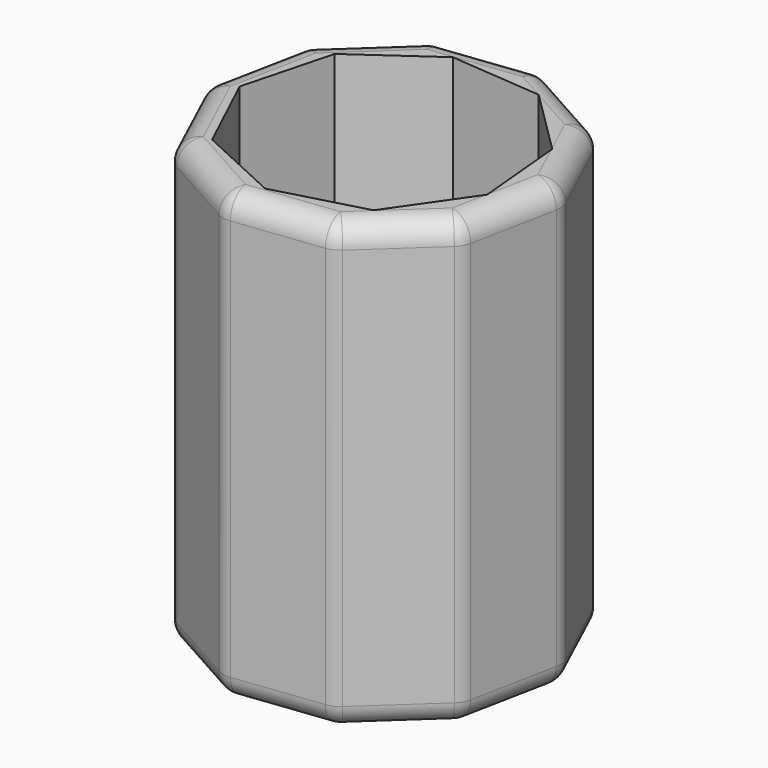
from build123d import *

# Parameters (mm, degrees)
F1_DEPTH      = 100
F2_T1_DEPTH   = 90
F2_T3_DEPTH   = 19.5857421182
F2_T5_DEPTH   = 19.5857421182
F2_T7_DEPTH   = 19.5857421182
F2_T9_DEPTH   = 19.5857421182
F2_T11_DEPTH  = 19.5857421182
F2_T13_DEPTH  = 19.5857421182
F2_T15_DEPTH  = 19.5857421182
F2_T17_DEPTH  = 19.5857421182
F2_T19_DEPTH  = 19.5857421182
F2_T21_DEPTH  = 19.5857421182
F2_T26_DEPTH  = 5
F2_T32_DEPTH  = 5
F2_T38_DEPTH  = 5
F2_T44_DEPTH  = 5
F2_T50_DEPTH  = 5
F2_T56_DEPTH  = 5
F2_T62_DEPTH  = 5
F2_T68_DEPTH  = 5
F2_T74_DEPTH  = 5
F2_T80_DEPTH  = 5
F2_T86_DEPTH  = 5
F2_T92_DEPTH  = 5
F2_T98_DEPTH  = 5
F2_T104_DEPTH = 5
F2_T110_DEPTH = 5
F2_T116_DEPTH = 5
F2_T122_DEPTH = 5
F2_T128_DEPTH = 5
F2_T134_DEPTH = 5
F2_T140_DEPTH = 5


# Not quite as in the source:
# - a fillet or chamfer that OpenCascade refuses, or shapes differently, is made with other operations: its cross-section is extruded or revolved along the edge and cut away or added


with BuildPart() as f1:
    # F0 (on Top) → F1 (new body)
    with BuildSketch(Plane.XY):
        Polygon((27.1144770649, 25.0985702318), (7.1835033032, 36.2426595944), (-15.491324562, 33.5432848347), (-32.2489929753, 18.0315153624), (-36.688642175, -4.3676801097), (-27.1144770649, -25.0985702318), (-7.1835033032, -36.2426595944), (15.491324562, -33.5432848347), (32.2489929753, -18.0315153624), (36.688642175, 4.3676801097), align=None)
        Polygon((-24.8698702516, 17.2562639713), (-7.9593132371, 29.2051095764), (12.675494899, 27.4885598321), (27.3792980994, 12.909807441), (29.272023432, -7.7095873283), (17.4680436786, -24.7215805041), (-2.5094278478, -30.1660714123), (-21.312710195, -21.4955222482), (-30.1435385776, -2.766979328), align=None, mode=Mode.SUBTRACT)
    extrude(amount=F1_DEPTH)

    # F2: fillet of radius 5 on 30 edges, made by hand

    # F2_s2 → F2_t1 (cut)
    with BuildSketch(Plane.XY.offset(5)):
        with BuildLine():
            ThreePointArc((-8.6014983146, -35.4498100673), (-7.1334759697, -35.9902585663), (-5.5702959817, -36.0506117803))
            Line((-5.5702959817, -36.0506117803), (-7.1835033032, -36.2426595944))
            Line((-7.1835033032, -36.2426595944), (-8.6014983146, -35.4498100673))
        make_face()
        with BuildLine():
            ThreePointArc((13.8781172405, -33.7353326487), (15.383439923, -33.3096827847), (16.6835538277, -32.4396954169))
            Line((16.6835538277, -32.4396954169), (15.491324562, -33.5432848347))
            Line((15.491324562, -33.5432848347), (13.8781172405, -33.7353326487))
        make_face()
        with BuildLine():
            ThreePointArc((32.5648531281, -16.4379179889), (32.024404629, -17.9059403338), (31.0567637096, -19.1351047802))
            Line((31.0567637096, -19.1351047802), (32.2489929753, -18.0315153624))
            Line((32.2489929753, -18.0315153624), (32.5648531281, -16.4379179889))
        make_face()
        with BuildLine():
            ThreePointArc((36.3727820222, 2.7740827361), (36.4331352362, 4.3372627241), (36.0074853722, 5.8425854066))
            Line((36.0074853722, 5.8425854066), (36.688642175, 4.3676801097))
            Line((36.688642175, 4.3676801097), (36.3727820222, 2.7740827361))
        make_face()
        with BuildLine():
            ThreePointArc((-27.7956338677, -23.6236649348), (-26.9256464999, -24.9237788395), (-25.6964820535, -25.8914197589))
            Line((-25.6964820535, -25.8914197589), (-27.1144770649, -25.0985702318))
            Line((-27.1144770649, -25.0985702318), (-27.7956338677, -23.6236649348))
        make_face()
        with BuildLine():
            ThreePointArc((-36.3727820222, -2.7740827361), (-36.4331352362, -4.3372627241), (-36.0074853722, -5.8425854066))
            Line((-36.0074853722, -5.8425854066), (-36.688642175, -4.3676801097))
            Line((-36.688642175, -4.3676801097), (-36.3727820222, -2.7740827361))
        make_face()
        with BuildLine():
            ThreePointArc((-31.0567637096, 19.1351047802), (-32.024404629, 17.9059403338), (-32.5648531281, 16.4379179889))
            Line((-32.5648531281, 16.4379179889), (-32.2489929753, 18.0315153624))
            Line((-32.2489929753, 18.0315153624), (-31.0567637096, 19.1351047802))
        make_face()
        with BuildLine():
            ThreePointArc((-13.8781172405, 33.7353326487), (-15.383439923, 33.3096827847), (-16.6835538277, 32.4396954169))
            Line((-16.6835538277, 32.4396954169), (-15.491324562, 33.5432848347))
            Line((-15.491324562, 33.5432848347), (-13.8781172405, 33.7353326487))
        make_face()
        with BuildLine():
            ThreePointArc((8.6014983146, 35.4498100673), (7.1334759697, 35.9902585663), (5.5702959817, 36.0506117803))
            Line((5.5702959817, 36.0506117803), (7.1835033032, 36.2426595944))
            Line((7.1835033032, 36.2426595944), (8.6014983146, 35.4498100673))
        make_face()
        with BuildLine():
            ThreePointArc((27.7956338677, 23.6236649348), (26.9256464999, 24.9237788395), (25.6964820535, 25.8914197589))
            Line((25.6964820535, 25.8914197589), (27.1144770649, 25.0985702318))
            Line((27.1144770649, 25.0985702318), (27.7956338677, 23.6236649348))
        make_face()
    extrude(amount=F2_T1_DEPTH, mode=Mode.SUBTRACT)

    # F2_s4 → F2_t3 (cut)
    with BuildSketch(Plane(origin=(-9.7242066111, -1.1576395658, 0), x_dir=(0, 0, 1), z_dir=(0.9929883231, 0.1182124791, 0))):
        with BuildLine():
            ThreePointArc((5, 35.1393580403), (1.4644660941, 33.6748919462), (0, 30.1393580403))
            Line((0, 30.1393580403), (0, 35.1393580403))
            Line((0, 35.1393580403), (5, 35.1393580403))
        make_face()
        with BuildLine():
            ThreePointArc((95, 35.1393580403), (98.5355339059, 33.6748919462), (100, 30.1393580403))
            Line((100, 30.1393580403), (100, 35.1393580403))
            Line((100, 35.1393580403), (95, 35.1393580403))
        make_face()
    extrude(amount=F2_T3_DEPTH, mode=Mode.SUBTRACT)

    # F2_s6 → F2_t5 (cut)
    with BuildSketch(Plane(origin=(-7.186604941, -6.6522953184, 0), x_dir=(0, 0, 1), z_dir=(0.7338608767, 0.6792997966, 0))):
        with BuildLine():
            ThreePointArc((5, 35.1393580403), (1.4644660941, 33.6748919462), (0, 30.1393580403))
            Line((0, 30.1393580403), (0, 35.1393580403))
            Line((0, 35.1393580403), (5, 35.1393580403))
        make_face()
        with BuildLine():
            ThreePointArc((95, 35.1393580403), (98.5355339059, 33.6748919462), (100, 30.1393580403))
            Line((100, 30.1393580403), (100, 35.1393580403))
            Line((100, 35.1393580403), (95, 35.1393580403))
        make_face()
    extrude(amount=F2_T5_DEPTH, mode=Mode.SUBTRACT)

    # F2_s8 → F2_t7 (cut)
    with BuildSketch(Plane(origin=(-1.9039644471, -9.6060003625, 0), x_dir=(0, 0, 1), z_dir=(0.1944235185, 0.9809176803, 0))):
        with BuildLine():
            ThreePointArc((5, 35.1393580403), (1.4644660941, 33.6748919462), (0, 30.1393580403))
            Line((0, 30.1393580403), (0, 35.1393580403))
            Line((0, 35.1393580403), (5, 35.1393580403))
        make_face()
        with BuildLine():
            ThreePointArc((95, 35.1393580403), (98.5355339059, 33.6748919462), (100, 30.1393580403))
            Line((100, 30.1393580403), (100, 35.1393580403))
            Line((100, 35.1393580403), (95, 35.1393580403))
        make_face()
    extrude(amount=F2_T7_DEPTH, mode=Mode.SUBTRACT)

    # F2_s10 → F2_t9 (cut)
    with BuildSketch(Plane(origin=(-8.5474918695, 4.7791951542, 0), x_dir=(0, 0, 1), z_dir=(0.8728279805, -0.4880279874, 0))):
        with BuildLine():
            ThreePointArc((5, 35.1393580403), (1.4644660941, 33.6748919462), (0, 30.1393580403))
            Line((0, 30.1393580403), (0, 35.1393580403))
            Line((0, 35.1393580403), (5, 35.1393580403))
        make_face()
        with BuildLine():
            ThreePointArc((95, 35.1393580403), (98.5355339059, 33.6748919462), (100, 30.1393580403))
            Line((100, 30.1393580403), (100, 35.1393580403))
            Line((100, 35.1393580403), (95, 35.1393580403))
        make_face()
    extrude(amount=F2_T9_DEPTH, mode=Mode.SUBTRACT)

    # F2_s12 → F2_t11 (cut)
    with BuildSketch(Plane(origin=(-4.1059257522, 8.8905397641, 0), x_dir=(0, 0, 1), z_dir=(0.4192770156, -0.9078583503, 0))):
        with BuildLine():
            ThreePointArc((5, 35.1393580403), (1.4644660941, 33.6748919462), (0, 30.1393580403))
            Line((0, 30.1393580403), (0, 35.1393580403))
            Line((0, 35.1393580403), (5, 35.1393580403))
        make_face()
        with BuildLine():
            ThreePointArc((95, 35.1393580403), (98.5355339059, 33.6748919462), (100, 30.1393580403))
            Line((100, 30.1393580403), (100, 35.1393580403))
            Line((100, 35.1393580403), (95, 35.1393580403))
        make_face()
    extrude(amount=F2_T11_DEPTH, mode=Mode.SUBTRACT)

    # F2_s14 → F2_t13 (cut)
    with BuildSketch(Plane(origin=(1.9039644471, 9.6060003625, 0), x_dir=(0, 0, 1), z_dir=(-0.1944235185, -0.9809176803, 0))):
        with BuildLine():
            ThreePointArc((5, 35.1393580403), (1.4644660941, 33.6748919462), (0, 30.1393580403))
            Line((0, 30.1393580403), (0, 35.1393580403))
            Line((0, 35.1393580403), (5, 35.1393580403))
        make_face()
        with BuildLine():
            ThreePointArc((95, 35.1393580403), (98.5355339059, 33.6748919462), (100, 30.1393580403))
            Line((100, 30.1393580403), (100, 35.1393580403))
            Line((100, 35.1393580403), (95, 35.1393580403))
        make_face()
    extrude(amount=F2_T13_DEPTH, mode=Mode.SUBTRACT)

    # F2_s16 → F2_t15 (cut)
    with BuildSketch(Plane(origin=(7.186604941, 6.6522953184, 0), x_dir=(0, 0, 1), z_dir=(-0.7338608767, -0.6792997966, 0))):
        with BuildLine():
            ThreePointArc((5, 35.1393580403), (1.4644660941, 33.6748919462), (0, 30.1393580403))
            Line((0, 30.1393580403), (0, 35.1393580403))
            Line((0, 35.1393580403), (5, 35.1393580403))
        make_face()
        with BuildLine():
            ThreePointArc((95, 35.1393580403), (98.5355339059, 33.6748919462), (100, 30.1393580403))
            Line((100, 30.1393580403), (100, 35.1393580403))
            Line((100, 35.1393580403), (95, 35.1393580403))
        make_face()
    extrude(amount=F2_T15_DEPTH, mode=Mode.SUBTRACT)

    # F2_s18 → F2_t17 (cut)
    with BuildSketch(Plane(origin=(9.7242066111, 1.1576395658, 0), x_dir=(0, 0, 1), z_dir=(-0.9929883231, -0.1182124791, 0))):
        with BuildLine():
            ThreePointArc((5, 35.1393580403), (1.4644660941, 33.6748919462), (0, 30.1393580403))
            Line((0, 30.1393580403), (0, 35.1393580403))
            Line((0, 35.1393580403), (5, 35.1393580403))
        make_face()
        with BuildLine():
            ThreePointArc((95, 35.1393580403), (98.5355339059, 33.6748919462), (100, 30.1393580403))
            Line((100, 30.1393580403), (100, 35.1393580403))
            Line((100, 35.1393580403), (95, 35.1393580403))
        make_face()
    extrude(amount=F2_T17_DEPTH, mode=Mode.SUBTRACT)

    # F2_s20 → F2_t19 (cut)
    with BuildSketch(Plane(origin=(8.5474918695, -4.7791951542, 0), x_dir=(0, 0, 1), z_dir=(-0.8728279805, 0.4880279874, 0))):
        with BuildLine():
            ThreePointArc((5, 35.1393580403), (1.4644660941, 33.6748919462), (0, 30.1393580403))
            Line((0, 30.1393580403), (0, 35.1393580403))
            Line((0, 35.1393580403), (5, 35.1393580403))
        make_face()
        with BuildLine():
            ThreePointArc((95, 35.1393580403), (98.5355339059, 33.6748919462), (100, 30.1393580403))
            Line((100, 30.1393580403), (100, 35.1393580403))
            Line((100, 35.1393580403), (95, 35.1393580403))
        make_face()
    extrude(amount=F2_T19_DEPTH, mode=Mode.SUBTRACT)

    # F2_s22 → F2_t21 (cut)
    with BuildSketch(Plane(origin=(4.1059257522, -8.8905397641, 0), x_dir=(0, 0, 1), z_dir=(-0.4192770156, 0.9078583503, 0))):
        with BuildLine():
            ThreePointArc((5, 35.1393580403), (1.4644660941, 33.6748919462), (0, 30.1393580403))
            Line((0, 30.1393580403), (0, 35.1393580403))
            Line((0, 35.1393580403), (5, 35.1393580403))
        make_face()
        with BuildLine():
            ThreePointArc((95, 35.1393580403), (98.5355339059, 33.6748919462), (100, 30.1393580403))
            Line((100, 30.1393580403), (100, 35.1393580403))
            Line((100, 35.1393580403), (95, 35.1393580403))
        make_face()
    extrude(amount=F2_T21_DEPTH, mode=Mode.SUBTRACT)


with BuildPart() as f2_tool24:
    # F2_s25 → F2_t26 (new body)
    with BuildSketch(Plane.XY.offset(5)):
        Polygon((-6.1613583774, -31.0856701649), (-8.6014983146, -35.4498100673), (-7.1835033032, -36.2426595944), (-5.5702959817, -36.0506117803), align=None)
    extrude(amount=-F2_T26_DEPTH)

    # F2_s27 → F2_t28 (revolve, cut)
    with BuildSketch(Plane(origin=(-6.1613583774, -31.0856701649, 5), x_dir=(0.1944235185, 0.9809176803, 0), z_dir=(-0.9809176803, 0.1944235185, 0))):
        with BuildLine():
            ThreePointArc((0, -5), (5, 0), (0, 5))
            Line((0, 5), (0, -5))
        make_face()
    revolve(axis=Axis((-6.1613583774, -31.0856701649, 5), (0, 0, -1)), mode=Mode.SUBTRACT)


with BuildPart() as f1_1:
    add(f1.part)

    # F2_t23: cut F2_tool24
    add(f2_tool24.part, mode=Mode.SUBTRACT)


with BuildPart() as f2_tool30:
    # F2_s31 → F2_t32 (new body)
    with BuildSketch(Plane.XY.offset(95)):
        Polygon((-6.1613583774, -31.0856701649), (-8.6014983146, -35.4498100673), (-7.1835033032, -36.2426595944), (-5.5702959817, -36.0506117803), align=None)
    extrude(amount=F2_T32_DEPTH)

    # F2_s33 → F2_t34 (revolve, cut)
    with BuildSketch(Plane(origin=(-6.1613583774, -31.0856701649, 95), x_dir=(0.1944235185, 0.9809176803, 0), z_dir=(0.9809176803, -0.1944235185, 0))):
        with BuildLine():
            ThreePointArc((0, -5), (5, 0), (0, 5))
            Line((0, 5), (0, -5))
        make_face()
    revolve(axis=Axis((-6.1613583774, -31.0856701649, 95), (0, 0, 1)), mode=Mode.SUBTRACT)


with BuildPart() as f1_2:
    add(f1_1.part)

    # F2_t29: cut F2_tool30
    add(f2_tool30.part, mode=Mode.SUBTRACT)


with BuildPart() as f2_tool36:
    # F2_s37 → F2_t38 (new body)
    with BuildSketch(Plane.XY.offset(5)):
        Polygon((13.2870548448, -28.7703910333), (13.8781172405, -33.7353326487), (15.491324562, -33.5432848347), (16.6835538277, -32.4396954169), align=None)
    extrude(amount=-F2_T38_DEPTH)

    # F2_s39 → F2_t40 (revolve, cut)
    with BuildSketch(Plane(origin=(13.2870548448, -28.7703910333, 5), x_dir=(-0.4192770156, 0.9078583503, 0), z_dir=(-0.9078583503, -0.4192770156, 0))):
        with BuildLine():
            ThreePointArc((0, -5), (5, 0), (0, 5))
            Line((0, 5), (0, -5))
        make_face()
    revolve(axis=Axis((13.2870548448, -28.7703910333, 5), (0, 0, -1)), mode=Mode.SUBTRACT)


with BuildPart() as f1_3:
    add(f1_2.part)

    # F2_t35: cut F2_tool36
    add(f2_tool36.part, mode=Mode.SUBTRACT)


with BuildPart() as f2_tool42:
    # F2_s43 → F2_t44 (new body)
    with BuildSketch(Plane.XY.offset(95)):
        Polygon((13.2870548448, -28.7703910333), (13.8781172405, -33.7353326487), (15.491324562, -33.5432848347), (16.6835538277, -32.4396954169), align=None)
    extrude(amount=F2_T44_DEPTH)

    # F2_s45 → F2_t46 (revolve, cut)
    with BuildSketch(Plane(origin=(13.2870548448, -28.7703910333, 95), x_dir=(-0.4192770156, 0.9078583503, 0), z_dir=(0.9078583503, 0.4192770156, 0))):
        with BuildLine():
            ThreePointArc((0, -5), (5, 0), (0, 5))
            Line((0, 5), (0, -5))
        make_face()
    revolve(axis=Axis((13.2870548448, -28.7703910333, 95), (0, 0, 1)), mode=Mode.SUBTRACT)


with BuildPart() as f1_4:
    add(f1_3.part)

    # F2_t41: cut F2_tool42
    add(f2_tool42.part, mode=Mode.SUBTRACT)


with BuildPart() as f2_tool48:
    # F2_s49 → F2_t50 (new body)
    with BuildSketch(Plane.XY.offset(5)):
        Polygon((27.6602647267, -15.4658003966), (32.5648531281, -16.4379179889), (32.2489929753, -18.0315153624), (31.0567637096, -19.1351047802), align=None)
    extrude(amount=-F2_T50_DEPTH)

    # F2_s51 → F2_t52 (revolve, cut)
    with BuildSketch(Plane(origin=(27.6602647267, -15.4658003966, 5), x_dir=(-0.8728279805, 0.4880279874, 0), z_dir=(-0.4880279874, -0.8728279805, 0))):
        with BuildLine():
            ThreePointArc((0, -5), (5, 0), (0, 5))
            Line((0, 5), (0, -5))
        make_face()
    revolve(axis=Axis((27.6602647267, -15.4658003966, 5), (0, 0, -1)), mode=Mode.SUBTRACT)


with BuildPart() as f1_5:
    add(f1_4.part)

    # F2_t47: cut F2_tool48
    add(f2_tool48.part, mode=Mode.SUBTRACT)


with BuildPart() as f2_tool54:
    # F2_s55 → F2_t56 (new body)
    with BuildSketch(Plane.XY.offset(95)):
        Polygon((27.6602647267, -15.4658003966), (32.5648531281, -16.4379179889), (32.2489929753, -18.0315153624), (31.0567637096, -19.1351047802), align=None)
    extrude(amount=F2_T56_DEPTH)

    # F2_s57 → F2_t58 (revolve, cut)
    with BuildSketch(Plane(origin=(27.6602647267, -15.4658003966, 95), x_dir=(-0.8728279805, 0.4880279874, 0), z_dir=(0.4880279874, 0.8728279805, 0))):
        with BuildLine():
            ThreePointArc((0, -5), (5, 0), (0, 5))
            Line((0, 5), (0, -5))
        make_face()
    revolve(axis=Axis((27.6602647267, -15.4658003966, 95), (0, 0, 1)), mode=Mode.SUBTRACT)


with BuildPart() as f1_6:
    add(f1_5.part)

    # F2_t53: cut F2_tool54
    add(f2_tool54.part, mode=Mode.SUBTRACT)


with BuildPart() as f2_tool60:
    # F2_s61 → F2_t62 (new body)
    with BuildSketch(Plane.XY.offset(5)):
        Polygon((31.4681936208, 3.7462003284), (36.3727820222, 2.7740827361), (36.688642175, 4.3676801097), (36.0074853722, 5.8425854066), align=None)
    extrude(amount=-F2_T62_DEPTH)

    # F2_s63 → F2_t64 (revolve, cut)
    with BuildSketch(Plane(origin=(31.4681936208, 3.7462003284, 5), x_dir=(-0.9929883231, -0.1182124791, 0), z_dir=(0.1182124791, -0.9929883231, 0))):
        with BuildLine():
            ThreePointArc((0, -5), (5, 0), (0, 5))
            Line((0, 5), (0, -5))
        make_face()
    revolve(axis=Axis((31.4681936208, 3.7462003284, 5), (0, 0, -1)), mode=Mode.SUBTRACT)


with BuildPart() as f1_7:
    add(f1_6.part)

    # F2_t59: cut F2_tool60
    add(f2_tool60.part, mode=Mode.SUBTRACT)


with BuildPart() as f2_tool66:
    # F2_s67 → F2_t68 (new body)
    with BuildSketch(Plane.XY.offset(95)):
        Polygon((31.4681936208, 3.7462003284), (36.3727820222, 2.7740827361), (36.688642175, 4.3676801097), (36.0074853722, 5.8425854066), align=None)
    extrude(amount=F2_T68_DEPTH)

    # F2_s69 → F2_t70 (revolve, cut)
    with BuildSketch(Plane(origin=(31.4681936208, 3.7462003284, 95), x_dir=(-0.9929883231, -0.1182124791, 0), z_dir=(-0.1182124791, 0.9929883231, 0))):
        with BuildLine():
            ThreePointArc((0, -5), (5, 0), (0, 5))
            Line((0, 5), (0, -5))
        make_face()
    revolve(axis=Axis((31.4681936208, 3.7462003284, 95), (0, 0, 1)), mode=Mode.SUBTRACT)


with BuildPart() as f1_8:
    add(f1_7.part)

    # F2_t65: cut F2_tool66
    add(f2_tool66.part, mode=Mode.SUBTRACT)


with BuildPart() as f2_tool72:
    # F2_s73 → F2_t74 (new body)
    with BuildSketch(Plane.XY.offset(5)):
        Polygon((-23.2563421164, -21.5272798566), (-27.7956338677, -23.6236649348), (-27.1144770649, -25.0985702318), (-25.6964820535, -25.8914197589), align=None)
    extrude(amount=-F2_T74_DEPTH)

    # F2_s75 → F2_t76 (revolve, cut)
    with BuildSketch(Plane(origin=(-23.2563421164, -21.5272798566, 5), x_dir=(0.7338608767, 0.6792997966, 0), z_dir=(-0.6792997966, 0.7338608767, 0))):
        with BuildLine():
            ThreePointArc((0, -5), (5, 0), (0, 5))
            Line((0, 5), (0, -5))
        make_face()
    revolve(axis=Axis((-23.2563421164, -21.5272798566, 5), (0, 0, -1)), mode=Mode.SUBTRACT)


with BuildPart() as f1_9:
    add(f1_8.part)

    # F2_t71: cut F2_tool72
    add(f2_tool72.part, mode=Mode.SUBTRACT)


with BuildPart() as f2_tool78:
    # F2_s79 → F2_t80 (new body)
    with BuildSketch(Plane.XY.offset(95)):
        Polygon((-23.2563421164, -21.5272798566), (-27.7956338677, -23.6236649348), (-27.1144770649, -25.0985702318), (-25.6964820535, -25.8914197589), align=None)
    extrude(amount=F2_T80_DEPTH)

    # F2_s81 → F2_t82 (revolve, cut)
    with BuildSketch(Plane(origin=(-23.2563421164, -21.5272798566, 95), x_dir=(0.7338608767, 0.6792997966, 0), z_dir=(0.6792997966, -0.7338608767, 0))):
        with BuildLine():
            ThreePointArc((0, -5), (5, 0), (0, 5))
            Line((0, 5), (0, -5))
        make_face()
    revolve(axis=Axis((-23.2563421164, -21.5272798566, 95), (0, 0, 1)), mode=Mode.SUBTRACT)


with BuildPart() as f1_10:
    add(f1_9.part)

    # F2_t77: cut F2_tool78
    add(f2_tool78.part, mode=Mode.SUBTRACT)


with BuildPart() as f2_tool84:
    # F2_s85 → F2_t86 (new body)
    with BuildSketch(Plane.XY.offset(5)):
        Polygon((-31.4681936208, -3.7462003284), (-36.3727820222, -2.7740827361), (-36.688642175, -4.3676801097), (-36.0074853722, -5.8425854066), align=None)
    extrude(amount=-F2_T86_DEPTH)

    # F2_s87 → F2_t88 (revolve, cut)
    with BuildSketch(Plane(origin=(-31.4681936208, -3.7462003284, 5), x_dir=(0.9929883231, 0.1182124791, 0), z_dir=(-0.1182124791, 0.9929883231, 0))):
        with BuildLine():
            ThreePointArc((0, -5), (5, 0), (0, 5))
            Line((0, 5), (0, -5))
        make_face()
    revolve(axis=Axis((-31.4681936208, -3.7462003284, 5), (0, 0, -1)), mode=Mode.SUBTRACT)


with BuildPart() as f1_11:
    add(f1_10.part)

    # F2_t83: cut F2_tool84
    add(f2_tool84.part, mode=Mode.SUBTRACT)


with BuildPart() as f2_tool90:
    # F2_s91 → F2_t92 (new body)
    with BuildSketch(Plane.XY.offset(95)):
        Polygon((-31.4681936208, -3.7462003284), (-36.3727820222, -2.7740827361), (-36.688642175, -4.3676801097), (-36.0074853722, -5.8425854066), align=None)
    extrude(amount=F2_T92_DEPTH)

    # F2_s93 → F2_t94 (revolve, cut)
    with BuildSketch(Plane(origin=(-31.4681936208, -3.7462003284, 95), x_dir=(0.9929883231, 0.1182124791, 0), z_dir=(0.1182124791, -0.9929883231, 0))):
        with BuildLine():
            ThreePointArc((0, -5), (5, 0), (0, 5))
            Line((0, 5), (0, -5))
        make_face()
    revolve(axis=Axis((-31.4681936208, -3.7462003284, 95), (0, 0, 1)), mode=Mode.SUBTRACT)


with BuildPart() as f1_12:
    add(f1_11.part)

    # F2_t89: cut F2_tool90
    add(f2_tool90.part, mode=Mode.SUBTRACT)


with BuildPart() as f2_tool96:
    # F2_s97 → F2_t98 (new body)
    with BuildSketch(Plane.XY.offset(5)):
        Polygon((-27.6602647267, 15.4658003966), (-31.0567637096, 19.1351047802), (-32.2489929753, 18.0315153624), (-32.5648531281, 16.4379179889), align=None)
    extrude(amount=-F2_T98_DEPTH)

    # F2_s99 → F2_t100 (revolve, cut)
    with BuildSketch(Plane(origin=(-27.6602647267, 15.4658003966, 5), x_dir=(0.8728279805, -0.4880279874, 0), z_dir=(0.4880279874, 0.8728279805, 0))):
        with BuildLine():
            ThreePointArc((0, -5), (5, 0), (0, 5))
            Line((0, 5), (0, -5))
        make_face()
    revolve(axis=Axis((-27.6602647267, 15.4658003966, 5), (0, 0, -1)), mode=Mode.SUBTRACT)


with BuildPart() as f1_13:
    add(f1_12.part)

    # F2_t95: cut F2_tool96
    add(f2_tool96.part, mode=Mode.SUBTRACT)


with BuildPart() as f2_tool102:
    # F2_s103 → F2_t104 (new body)
    with BuildSketch(Plane.XY.offset(95)):
        Polygon((-27.6602647267, 15.4658003966), (-31.0567637096, 19.1351047802), (-32.2489929753, 18.0315153624), (-32.5648531281, 16.4379179889), align=None)
    extrude(amount=F2_T104_DEPTH)

    # F2_s105 → F2_t106 (revolve, cut)
    with BuildSketch(Plane(origin=(-27.6602647267, 15.4658003966, 95), x_dir=(0.8728279805, -0.4880279874, 0), z_dir=(-0.4880279874, -0.8728279805, 0))):
        with BuildLine():
            ThreePointArc((0, -5), (5, 0), (0, 5))
            Line((0, 5), (0, -5))
        make_face()
    revolve(axis=Axis((-27.6602647267, 15.4658003966, 95), (0, 0, 1)), mode=Mode.SUBTRACT)


with BuildPart() as f1_14:
    add(f1_13.part)

    # F2_t101: cut F2_tool102
    add(f2_tool102.part, mode=Mode.SUBTRACT)


with BuildPart() as f2_tool108:
    # F2_s109 → F2_t110 (new body)
    with BuildSketch(Plane.XY.offset(5)):
        Polygon((-13.2870548448, 28.7703910333), (-13.8781172405, 33.7353326487), (-15.491324562, 33.5432848347), (-16.6835538277, 32.4396954169), align=None)
    extrude(amount=-F2_T110_DEPTH)

    # F2_s111 → F2_t112 (revolve, cut)
    with BuildSketch(Plane(origin=(-13.2870548448, 28.7703910333, 5), x_dir=(0.4192770156, -0.9078583503, 0), z_dir=(0.9078583503, 0.4192770156, 0))):
        with BuildLine():
            ThreePointArc((0, -5), (5, 0), (0, 5))
            Line((0, 5), (0, -5))
        make_face()
    revolve(axis=Axis((-13.2870548448, 28.7703910333, 5), (0, 0, -1)), mode=Mode.SUBTRACT)


with BuildPart() as f1_15:
    add(f1_14.part)

    # F2_t107: cut F2_tool108
    add(f2_tool108.part, mode=Mode.SUBTRACT)


with BuildPart() as f2_tool114:
    # F2_s115 → F2_t116 (new body)
    with BuildSketch(Plane.XY.offset(95)):
        Polygon((-13.2870548448, 28.7703910333), (-13.8781172405, 33.7353326487), (-15.491324562, 33.5432848347), (-16.6835538277, 32.4396954169), align=None)
    extrude(amount=F2_T116_DEPTH)

    # F2_s117 → F2_t118 (revolve, cut)
    with BuildSketch(Plane(origin=(-13.2870548448, 28.7703910333, 95), x_dir=(0.4192770156, -0.9078583503, 0), z_dir=(-0.9078583503, -0.4192770156, 0))):
        with BuildLine():
            ThreePointArc((0, -5), (5, 0), (0, 5))
            Line((0, 5), (0, -5))
        make_face()
    revolve(axis=Axis((-13.2870548448, 28.7703910333, 95), (0, 0, 1)), mode=Mode.SUBTRACT)


with BuildPart() as f1_16:
    add(f1_15.part)

    # F2_t113: cut F2_tool114
    add(f2_tool114.part, mode=Mode.SUBTRACT)


with BuildPart() as f2_tool120:
    # F2_s121 → F2_t122 (new body)
    with BuildSketch(Plane.XY.offset(5)):
        Polygon((6.1613583774, 31.0856701649), (8.6014983146, 35.4498100673), (7.1835033032, 36.2426595944), (5.5702959817, 36.0506117803), align=None)
    extrude(amount=-F2_T122_DEPTH)

    # F2_s123 → F2_t124 (revolve, cut)
    with BuildSketch(Plane(origin=(6.1613583774, 31.0856701649, 5), x_dir=(-0.1944235185, -0.9809176803, 0), z_dir=(0.9809176803, -0.1944235185, 0))):
        with BuildLine():
            ThreePointArc((0, -5), (5, 0), (0, 5))
            Line((0, 5), (0, -5))
        make_face()
    revolve(axis=Axis((6.1613583774, 31.0856701649, 5), (0, 0, -1)), mode=Mode.SUBTRACT)


with BuildPart() as f1_17:
    add(f1_16.part)

    # F2_t119: cut F2_tool120
    add(f2_tool120.part, mode=Mode.SUBTRACT)


with BuildPart() as f2_tool126:
    # F2_s127 → F2_t128 (new body)
    with BuildSketch(Plane.XY.offset(95)):
        Polygon((6.1613583774, 31.0856701649), (8.6014983146, 35.4498100673), (7.1835033032, 36.2426595944), (5.5702959817, 36.0506117803), align=None)
    extrude(amount=F2_T128_DEPTH)

    # F2_s129 → F2_t130 (revolve, cut)
    with BuildSketch(Plane(origin=(6.1613583774, 31.0856701649, 95), x_dir=(-0.1944235185, -0.9809176803, 0), z_dir=(-0.9809176803, 0.1944235185, 0))):
        with BuildLine():
            ThreePointArc((0, -5), (5, 0), (0, 5))
            Line((0, 5), (0, -5))
        make_face()
    revolve(axis=Axis((6.1613583774, 31.0856701649, 95), (0, 0, 1)), mode=Mode.SUBTRACT)


with BuildPart() as f1_18:
    add(f1_17.part)

    # F2_t125: cut F2_tool126
    add(f2_tool126.part, mode=Mode.SUBTRACT)


with BuildPart() as f2_tool132:
    # F2_s133 → F2_t134 (new body)
    with BuildSketch(Plane.XY.offset(5)):
        Polygon((23.2563421164, 21.5272798566), (27.7956338677, 23.6236649348), (27.1144770649, 25.0985702318), (25.6964820535, 25.8914197589), align=None)
    extrude(amount=-F2_T134_DEPTH)

    # F2_s135 → F2_t136 (revolve, cut)
    with BuildSketch(Plane(origin=(23.2563421164, 21.5272798566, 5), x_dir=(-0.7338608767, -0.6792997966, 0), z_dir=(0.6792997966, -0.7338608767, 0))):
        with BuildLine():
            ThreePointArc((0, -5), (5, 0), (0, 5))
            Line((0, 5), (0, -5))
        make_face()
    revolve(axis=Axis((23.2563421164, 21.5272798566, 5), (0, 0, -1)), mode=Mode.SUBTRACT)


with BuildPart() as f1_19:
    add(f1_18.part)

    # F2_t131: cut F2_tool132
    add(f2_tool132.part, mode=Mode.SUBTRACT)


with BuildPart() as f2_tool138:
    # F2_s139 → F2_t140 (new body)
    with BuildSketch(Plane.XY.offset(95)):
        Polygon((23.2563421164, 21.5272798566), (27.7956338677, 23.6236649348), (27.1144770649, 25.0985702318), (25.6964820535, 25.8914197589), align=None)
    extrude(amount=F2_T140_DEPTH)

    # F2_s141 → F2_t142 (revolve, cut)
    with BuildSketch(Plane(origin=(23.2563421164, 21.5272798566, 95), x_dir=(-0.7338608767, -0.6792997966, 0), z_dir=(-0.6792997966, 0.7338608767, 0))):
        with BuildLine():
            ThreePointArc((0, -5), (5, 0), (0, 5))
            Line((0, 5), (0, -5))
        make_face()
    revolve(axis=Axis((23.2563421164, 21.5272798566, 95), (0, 0, 1)), mode=Mode.SUBTRACT)


with BuildPart() as f1_20:
    add(f1_19.part)

    # F2_t137: cut F2_tool138
    add(f2_tool138.part, mode=Mode.SUBTRACT)


solid = f1_20.part
